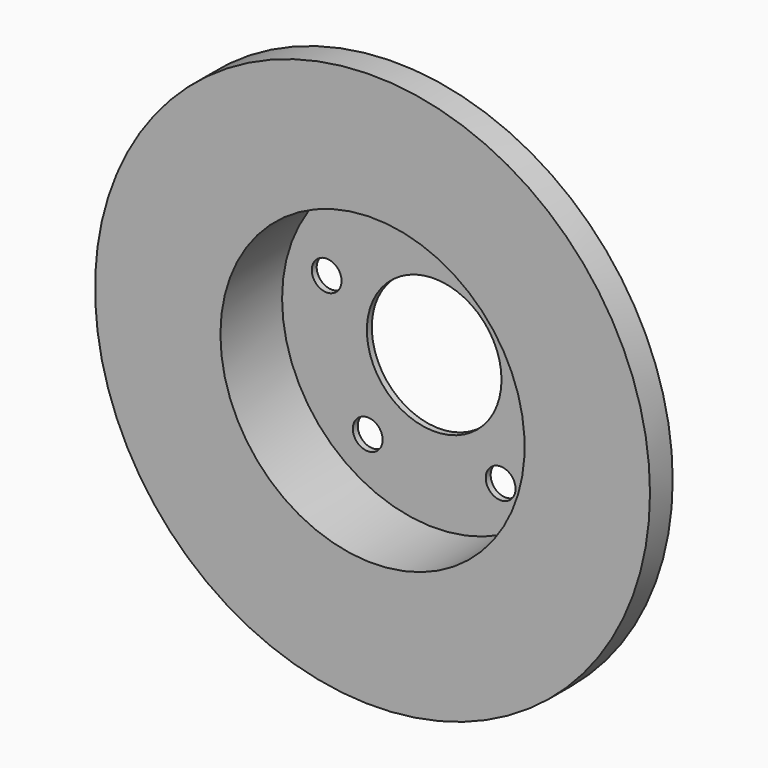
from build123d import *

# Parameters (mm, degrees)
F0_R     = 74
F0_R_2   = 7.25
F0_R_3   = 32.75
F1_DEPTH = 3
F2_R     = 81
F2_R_2   = 74
F3_DEPTH = 40.5
F4_R     = 135
F4_R_2   = 81
F5_DEPTH = 13.8


with BuildPart() as f1:
    # F0 (on Front) → F1 (new body)
    with BuildSketch(Plane.XZ):
        Circle(F0_R)
        with Locations((-32.3281888761, -44.4959346906)):
            Circle(F0_R_2, mode=Mode.SUBTRACT)
        with Locations((32.3281888761, -44.4959346906)):
            Circle(F0_R_2, mode=Mode.SUBTRACT)
        with Locations((-52.3081083962, 16.9959346906)):
            Circle(F0_R_2, mode=Mode.SUBTRACT)
        Circle(F0_R_3, mode=Mode.SUBTRACT)
        with Locations((52.3081083962, 16.9959346906)):
            Circle(F0_R_2, mode=Mode.SUBTRACT)
        with Locations((0, 55)):
            Circle(F0_R_2, mode=Mode.SUBTRACT)
    extrude(amount=F1_DEPTH)

    # F2 (on face) → F3 (join)
    with BuildSketch(Plane(origin=(0, 0, 0), x_dir=(-1, 0, 0), z_dir=(0, 1, 0))):
        Circle(F2_R)
        Circle(F2_R_2, mode=Mode.SUBTRACT)
    extrude(amount=-F3_DEPTH)

    # F4 (on face) → F5 (join)
    with BuildSketch(Plane.XZ.offset(40.5)):
        Circle(F4_R)
        Circle(F4_R_2, mode=Mode.SUBTRACT)
    extrude(amount=-F5_DEPTH)


solid = f1.part
